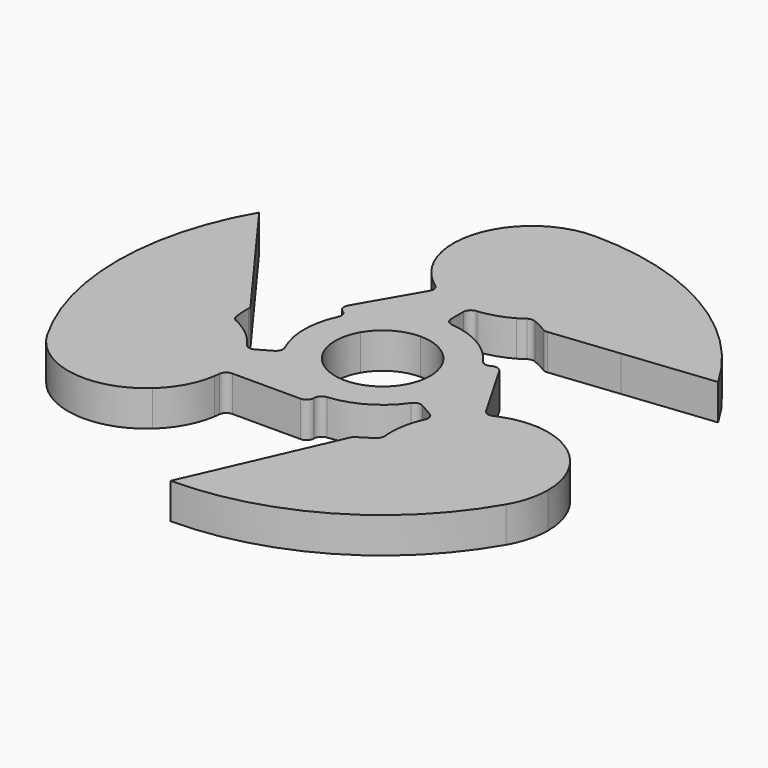
from build123d import *

# Parameters (mm, degrees)
F1_DEPTH = 4.7625
F2_R     = 1


with BuildPart() as f1:
    # F0 (on Top) → F1 (new body)
    with BuildSketch(Plane.XY):
        with BuildLine():
            ThreePointArc((-5.499261314, -3.175), (-6.35, 0), (-5.499261314, 3.175))
            Line((-5.499261314, 3.175), (-9.0932667397, 5.25))
            ThreePointArc((-9.0932667397, 5.25), (-10.5, 0), (-9.0932667397, -5.25))
            Line((-9.0932667397, -5.25), (-5.499261314, -3.175))
        make_face()
        with BuildLine():
            Line((0, -10.5), (0, -6.35))
            ThreePointArc((0, -6.35), (-3.175, -5.499261314), (-5.499261314, -3.175))
            Line((-5.499261314, -3.175), (-9.0932667397, -5.25))
            ThreePointArc((-9.0932667397, -5.25), (-5.25, -9.0932667397), (0, -10.5))
        make_face()
        with BuildLine():
            Line((9.0932667397, -5.25), (5.499261314, -3.175))
            ThreePointArc((5.499261314, -3.175), (3.175, -5.499261314), (0, -6.35))
            Line((0, -6.35), (0, -10.5))
            ThreePointArc((0, -10.5), (5.25, -9.0932667397), (9.0932667397, -5.25))
        make_face()
        with BuildLine():
            ThreePointArc((5.499261314, 3.175), (6.1336289969, 1.6435009364), (6.35, 0))
            ThreePointArc((6.35, 0), (6.1336289969, -1.6435009364), (5.499261314, -3.175))
            Line((5.499261314, -3.175), (9.0932667397, -5.25))
            ThreePointArc((9.0932667397, -5.25), (10.142221176, -2.7175999736), (10.5, 0))
            ThreePointArc((10.5, 0), (10.142221176, 2.7175999736), (9.0932667397, 5.25))
            Line((9.0932667397, 5.25), (5.499261314, 3.175))
        make_face()
        with BuildLine():
            ThreePointArc((0, 6.35), (3.175, 5.499261314), (5.499261314, 3.175))
            Line((5.499261314, 3.175), (9.0932667397, 5.25))
            ThreePointArc((9.0932667397, 5.25), (5.25, 9.0932667397), (0, 10.5))
            Line((0, 10.5), (0, 6.35))
        make_face()
        with BuildLine():
            ThreePointArc((-5.499261314, 3.175), (-3.175, 5.499261314), (0, 6.35))
            Line((0, 6.35), (0, 10.5))
            ThreePointArc((0, 10.5), (-5.25, 9.0932667397), (-9.0932667397, 5.25))
            Line((-9.0932667397, 5.25), (-5.499261314, 3.175))
        make_face()
        with BuildLine():
            Line((-30.6832667397, -17.7149923118), (-21.59, -12.4649923118))
            ThreePointArc((-21.59, -12.4649923118), (-23.7308339091, -7.638825519), (-24.8073171849, -2.4700500843))
            ThreePointArc((-24.8073171849, -2.4700500843), (-31.387432573, -8.6887090891), (-30.6832667397, -17.7149923118))
        make_face()
        with BuildLine():
            ThreePointArc((-14.5427847141, -20.2487418398), (-18.4808339091, -16.7320922588), (-21.59, -12.4649923118))
            Line((-21.59, -12.4649923118), (-30.6832667397, -17.7149923118))
            ThreePointArc((-30.6832667397, -17.7149923118), (-23.2183590837, -22.8379594232), (-14.5427847141, -20.2487418398))
        make_face()
        with BuildLine():
            ThreePointArc((-24.8073171849, -2.4700500843), (-24.7664239313, 2.8510312146), (-23.5971783755, 8.0422202188))
            Line((-23.5971783755, 8.0422202188), (-30.6832667397, 17.7149923118))
            ThreePointArc((-30.6832667397, 17.7149923118), (-35.4299846236, 0), (-30.6832667397, -17.7149923118))
            ThreePointArc((-30.6832667397, -17.7149923118), (-31.387432573, -8.6887090891), (-24.8073171849, -2.4700500843))
        make_face()
        with BuildLine():
            ThreePointArc((-17.8004721403, -2.6726749865), (-17.9637015789, -1.1425522236), (-17.9956452163, 0.3959207605))
            Line((-17.9956452163, 0.3959207605), (-23.5971783755, 8.0422202188))
            ThreePointArc((-23.5971783755, 8.0422202188), (-24.7664239313, 2.8510312146), (-24.8073171849, -2.4700500843))
            ThreePointArc((-24.8073171849, -2.4700500843), (-21.286486447, -1.9693799179), (-17.8004721403, -2.6726749865))
        make_face()
        with BuildLine():
            Line((-21.59, -12.4649923118), (-17.2877645627, -5.0133019483))
            ThreePointArc((-17.2877645627, -5.0133019483), (-17.5831090076, -3.851529258), (-17.8004721403, -2.6726749865))
            ThreePointArc((-17.8004721403, -2.6726749865), (-21.286486447, -1.9693799179), (-24.8073171849, -2.4700500843))
            ThreePointArc((-24.8073171849, -2.4700500843), (-23.7308339091, -7.638825519), (-21.59, -12.4649923118))
        make_face()
        with BuildLine():
            ThreePointArc((-11.2148405045, -14.0793235796), (-12.1270766847, -13.3016544491), (-12.9855291254, -12.4649923118))
            Line((-12.9855291254, -12.4649923118), (-21.59, -12.4649923118))
            ThreePointArc((-21.59, -12.4649923118), (-18.4808339091, -16.7320922588), (-14.5427847141, -20.2487418398))
            ThreePointArc((-14.5427847141, -20.2487418398), (-12.3487762621, -17.4499480615), (-11.2148405045, -14.0793235796))
        make_face()
        with BuildLine():
            ThreePointArc((-12.9855291254, -12.4649923118), (-14.3916544405, -10.8111184651), (-15.5884572681, -9))
            Line((-15.5884572681, -9), (-21.59, -12.4649923118))
            Line((-21.59, -12.4649923118), (-12.9855291254, -12.4649923118))
        make_face()
        with BuildLine():
            Line((-21.59, -12.4649923118), (-15.5884572681, -9))
            ThreePointArc((-15.5884572681, -9), (-16.5585304543, -7.0579791154), (-17.2877645627, -5.0133019483))
            Line((-17.2877645627, -5.0133019483), (-21.59, -12.4649923118))
        make_face()
        with BuildLine():
            Line((-15.5884572681, -9), (-12.4967332603, -7.2149923118))
            ThreePointArc((-12.4967332603, -7.2149923118), (-12.8045182874, -6.7147478755), (-13.139793395, -6.2324961559))
            ThreePointArc((-13.139793395, -6.2324961559), (-14.5921490915, -4.6368327157), (-16.34, -3.3717255721))
            Line((-16.34, -3.3717255721), (-17.2877645627, -5.0133019483))
            ThreePointArc((-17.2877645627, -5.0133019483), (-16.5585304543, -7.0579791154), (-15.5884572681, -9))
        make_face()
        with BuildLine():
            ThreePointArc((-11.09, -12.4649923118), (-11.447778824, -9.7473923382), (-12.4967332603, -7.2149923118))
            Line((-12.4967332603, -7.2149923118), (-15.5884572681, -9))
            ThreePointArc((-15.5884572681, -9), (-14.3916544405, -10.8111184651), (-12.9855291254, -12.4649923118))
            Line((-12.9855291254, -12.4649923118), (-11.09, -12.4649923118))
        make_face()
        with BuildLine():
            Line((-17.2877645627, -5.0133019483), (-16.34, -3.3717255721))
            ThreePointArc((-16.34, -3.3717255721), (-17.0567413584, -2.9940068252), (-17.8004721403, -2.6726749865))
            ThreePointArc((-17.8004721403, -2.6726749865), (-17.5831090076, -3.851529258), (-17.2877645627, -5.0133019483))
        make_face()
        with BuildLine():
            ThreePointArc((-11.2148405045, -14.0793235796), (-11.1212566489, -13.2745679095), (-11.09, -12.4649923118))
            Line((-11.09, -12.4649923118), (-12.9855291254, -12.4649923118))
            ThreePointArc((-12.9855291254, -12.4649923118), (-12.1270766847, -13.3016544491), (-11.2148405045, -14.0793235796))
        make_face()
        with BuildLine():
            Line((21.59, -12.4649923118), (17.2877645627, -5.0133019483))
            ThreePointArc((17.2877645627, -5.0133019483), (16.5585304543, -7.0579791154), (15.5884572681, -9))
            Line((15.5884572681, -9), (21.59, -12.4649923118))
        make_face()
        with BuildLine():
            Line((17.2877645627, -5.0133019483), (16.34, -3.3717255721))
            ThreePointArc((16.34, -3.3717255721), (14.1653787975, -5.0403711093), (12.4967332603, -7.2149923118))
            Line((12.4967332603, -7.2149923118), (15.5884572681, -9))
            ThreePointArc((15.5884572681, -9), (16.5585304543, -7.0579791154), (17.2877645627, -5.0133019483))
        make_face()
        with BuildLine():
            Line((15.5884572681, -9), (12.4967332603, -7.2149923118))
            ThreePointArc((12.4967332603, -7.2149923118), (12.2250524559, -7.7165444079), (11.9810090739, -8.2321099153))
            ThreePointArc((11.9810090739, -8.2321099153), (11.3151665531, -10.3021706275), (11.09, -12.4649923118))
            Line((11.09, -12.4649923118), (12.9855291254, -12.4649923118))
            ThreePointArc((12.9855291254, -12.4649923118), (14.3916544405, -10.8111184651), (15.5884572681, -9))
        make_face()
        with BuildLine():
            Line((21.59, -12.4649923118), (15.5884572681, -9))
            ThreePointArc((15.5884572681, -9), (14.3916544405, -10.8111184651), (12.9855291254, -12.4649923118))
            Line((12.9855291254, -12.4649923118), (21.59, -12.4649923118))
        make_face()
        with BuildLine():
            ThreePointArc((14.5427847141, -20.2487418398), (18.4808339091, -16.7320922588), (21.59, -12.4649923118))
            Line((21.59, -12.4649923118), (12.9855291254, -12.4649923118))
            ThreePointArc((12.9855291254, -12.4649923118), (12.1270766847, -13.3016544491), (11.2148405045, -14.0793235796))
            ThreePointArc((11.2148405045, -14.0793235796), (12.3487762621, -17.4499480615), (14.5427847141, -20.2487418398))
        make_face()
        with BuildLine():
            ThreePointArc((24.8073171849, -2.4700500843), (23.7308339091, -7.638825519), (21.59, -12.4649923118))
            Line((21.59, -12.4649923118), (30.6832667397, -17.7149923118))
            ThreePointArc((30.6832667397, -17.7149923118), (31.732221176, -15.1825922854), (32.09, -12.4649923118))
            ThreePointArc((32.09, -12.4649923118), (30.0762191358, -6.2816206766), (24.8073171849, -2.4700500843))
        make_face()
        with BuildLine():
            ThreePointArc((17.8004721403, -2.6726749865), (17.5831090076, -3.851529258), (17.2877645627, -5.0133019483))
            Line((17.2877645627, -5.0133019483), (21.59, -12.4649923118))
            ThreePointArc((21.59, -12.4649923118), (23.7308339091, -7.638825519), (24.8073171849, -2.4700500843))
            ThreePointArc((24.8073171849, -2.4700500843), (21.286486447, -1.9693799179), (17.8004721403, -2.6726749865))
        make_face()
        with BuildLine():
            ThreePointArc((17.8004721403, -2.6726749865), (17.0567413584, -2.9940068252), (16.34, -3.3717255721))
            Line((16.34, -3.3717255721), (17.2877645627, -5.0133019483))
            ThreePointArc((17.2877645627, -5.0133019483), (17.5831090076, -3.851529258), (17.8004721403, -2.6726749865))
        make_face()
        with BuildLine():
            ThreePointArc((30.6832667397, -17.7149923118), (23.2183590837, -22.8379594232), (14.5427847141, -20.2487418398))
            ThreePointArc((14.5427847141, -20.2487418398), (9.9141341412, -22.8738732523), (4.8337957326, -24.4568712666))
            Line((4.8337957326, -24.4568712666), (0, -35.4299846236))
            ThreePointArc((0, -35.4299846236), (17.7149923118, -30.6832667397), (30.6832667397, -17.7149923118))
        make_face()
        with BuildLine():
            ThreePointArc((11.2148405045, -14.0793235796), (9.9713029836, -14.9857638047), (8.6548881807, -15.7826775479))
            Line((8.6548881807, -15.7826775479), (4.8337957326, -24.4568712666))
            ThreePointArc((4.8337957326, -24.4568712666), (9.9141341412, -22.8738732523), (14.5427847141, -20.2487418398))
            ThreePointArc((14.5427847141, -20.2487418398), (12.3487762621, -17.4499480615), (11.2148405045, -14.0793235796))
        make_face()
        with BuildLine():
            Line((12.9855291254, -12.4649923118), (11.09, -12.4649923118))
            ThreePointArc((11.09, -12.4649923118), (11.1212566489, -13.2745679095), (11.2148405045, -14.0793235796))
            ThreePointArc((11.2148405045, -14.0793235796), (12.1270766847, -13.3016544491), (12.9855291254, -12.4649923118))
        make_face()
        with BuildLine():
            Line((30.6832667397, -17.7149923118), (21.59, -12.4649923118))
            ThreePointArc((21.59, -12.4649923118), (18.4808339091, -16.7320922588), (14.5427847141, -20.2487418398))
            ThreePointArc((14.5427847141, -20.2487418398), (23.2183590837, -22.8379594232), (30.6832667397, -17.7149923118))
        make_face()
        with BuildLine():
            Line((0, 18), (0, 14.4299846236))
            ThreePointArc((0, 14.4299846236), (0.5701972901, 14.4454781951), (1.1387118387, 14.4919131854))
            ThreePointArc((1.1387118387, 14.4919131854), (3.2643582308, 14.9503070065), (5.25, 15.8367178839))
            Line((5.25, 15.8367178839), (4.3022354373, 17.4782942601))
            ThreePointArc((4.3022354373, 17.4782942601), (2.1668760138, 17.8690975805), (0, 18))
        make_face()
        with BuildLine():
            ThreePointArc((-4.3022354373, 17.4782942601), (-2.1668760138, 17.8690975805), (0, 18))
            Line((0, 18), (0, 24.9299846236))
            Line((0, 24.9299846236), (-4.3022354373, 17.4782942601))
        make_face()
        with BuildLine():
            Line((0, 24.9299846236), (0, 18))
            ThreePointArc((0, 18), (2.1668760138, 17.8690975805), (4.3022354373, 17.4782942601))
            Line((4.3022354373, 17.4782942601), (0, 24.9299846236))
        make_face()
        with BuildLine():
            ThreePointArc((-6.5856316358, 16.7519985661), (-5.9354847095, 16.2685747347), (-5.25, 15.8367178839))
            Line((-5.25, 15.8367178839), (-4.3022354373, 17.4782942601))
            ThreePointArc((-4.3022354373, 17.4782942601), (-5.456032323, 17.1531837071), (-6.5856316358, 16.7519985661))
        make_face()
        with BuildLine():
            Line((0, 24.9299846236), (4.3022354373, 17.4782942601))
            ThreePointArc((4.3022354373, 17.4782942601), (5.456032323, 17.1531837071), (6.5856316358, 16.7519985661))
            ThreePointArc((6.5856316358, 16.7519985661), (8.9377101849, 19.4193279794), (10.2645324709, 22.718791924))
            ThreePointArc((10.2645324709, 22.718791924), (5.25, 24.3709177778), (0, 24.9299846236))
        make_face()
        with BuildLine():
            Line((4.3022354373, 17.4782942601), (5.25, 15.8367178839))
            ThreePointArc((5.25, 15.8367178839), (5.9354847095, 16.2685747347), (6.5856316358, 16.7519985661))
            ThreePointArc((6.5856316358, 16.7519985661), (5.456032323, 17.1531837071), (4.3022354373, 17.4782942601))
        make_face()
        with BuildLine():
            ThreePointArc((-5.25, 15.8367178839), (-2.7175999736, 14.7877634476), (0, 14.4299846236))
            Line((0, 14.4299846236), (0, 18))
            ThreePointArc((0, 18), (-2.1668760138, 17.8690975805), (-4.3022354373, 17.4782942601))
            Line((-4.3022354373, 17.4782942601), (-5.25, 15.8367178839))
        make_face()
        with BuildLine():
            ThreePointArc((-6.5856316358, 16.7519985661), (-5.456032323, 17.1531837071), (-4.3022354373, 17.4782942601))
            Line((-4.3022354373, 17.4782942601), (0, 24.9299846236))
            ThreePointArc((0, 24.9299846236), (-5.25, 24.3709177778), (-10.2645324709, 22.718791924))
            ThreePointArc((-10.2645324709, 22.718791924), (-8.9377101849, 19.4193279794), (-6.5856316358, 16.7519985661))
        make_face()
        with BuildLine():
            ThreePointArc((-10.2645324709, 22.718791924), (-5.25, 24.3709177778), (0, 24.9299846236))
            Line((0, 24.9299846236), (0, 35.4299846236))
            ThreePointArc((0, 35.4299846236), (-8.1690734892, 31.5266685123), (-10.2645324709, 22.718791924))
        make_face()
        with BuildLine():
            Line((0, 35.4299846236), (0, 24.9299846236))
            ThreePointArc((0, 24.9299846236), (5.25, 24.3709177778), (10.2645324709, 22.718791924))
            ThreePointArc((10.2645324709, 22.718791924), (10.4409671713, 23.8181372744), (10.5, 24.9299846236))
            ThreePointArc((10.5, 24.9299846236), (7.4246212025, 32.3546058261), (0, 35.4299846236))
        make_face()
        with BuildLine():
            ThreePointArc((10.2645324709, 22.718791924), (14.8522882489, 20.022828649), (18.7633739476, 16.4146255344))
            Line((18.7633739476, 16.4146255344), (30.6832667397, 17.7149923118))
            ThreePointArc((30.6832667397, 17.7149923118), (17.7149923118, 30.6832667397), (0, 35.4299846236))
            ThreePointArc((0, 35.4299846236), (7.4246212025, 32.3546058261), (10.5, 24.9299846236))
            ThreePointArc((10.5, 24.9299846236), (10.4409671713, 23.8181372744), (10.2645324709, 22.718791924))
        make_face()
        with BuildLine():
            ThreePointArc((6.5856316358, 16.7519985661), (7.9924006582, 16.128283595), (9.3407556058, 15.3866918053))
            Line((9.3407556058, 15.3866918053), (18.7633739476, 16.4146255344))
            ThreePointArc((18.7633739476, 16.4146255344), (14.8522882489, 20.022828649), (10.2645324709, 22.718791924))
            ThreePointArc((10.2645324709, 22.718791924), (8.9377101849, 19.4193279794), (6.5856316358, 16.7519985661))
        make_face()
        with BuildLine():
            ThreePointArc((-9.0932667397, 5.25), (-5.25, 9.0932667397), (0, 10.5))
            Line((0, 10.5), (0, 14.3676886584))
            Line((0, 14.3676886584), (0, 14.4299846236))
            ThreePointArc((0, 14.4299846236), (-2.7175999736, 14.7877634476), (-5.25, 15.8367178839))
            Line((-5.25, 15.8367178839), (-10.795, 6.2324961559))
            Line((-10.795, 6.2324961559), (-9.0932667397, 5.25))
        make_face()
        with BuildLine():
            Line((10.795, 6.2324961559), (9.0932667397, 5.25))
            ThreePointArc((9.0932667397, 5.25), (10.142221176, 2.7175999736), (10.5, 0))
            ThreePointArc((10.5, 0), (10.142221176, -2.7175999736), (9.0932667397, -5.25))
            Line((9.0932667397, -5.25), (12.4427833719, -7.1838443292))
            Line((12.4427833719, -7.1838443292), (12.4967332603, -7.2149923118))
            ThreePointArc((12.4967332603, -7.2149923118), (14.1653787975, -5.0403711093), (16.34, -3.3717255721))
            Line((16.34, -3.3717255721), (10.795, 6.2324961559))
        make_face()
        with BuildLine():
            Line((0, -12.4649923118), (0, -10.5))
            ThreePointArc((0, -10.5), (-5.25, -9.0932667397), (-9.0932667397, -5.25))
            Line((-9.0932667397, -5.25), (-12.4967332603, -7.2149923118))
            ThreePointArc((-12.4967332603, -7.2149923118), (-11.447778824, -9.7473923382), (-11.09, -12.4649923118))
            Line((-11.09, -12.4649923118), (0, -12.4649923118))
        make_face()
    extrude(amount=F1_DEPTH)

    # F2
    f2_edges = [f1.edges().sort_by_distance(p)[0] for p in [
        (0, -12.464992, 2.38125),
        (10.795, 6.232496, 2.38125),
        (-10.795, 6.232496, 2.38125),
        (8.654888, -15.782678, 2.38125),
        (11.214841, -14.079324, 2.38125),
        (-17.995645, 0.395921, 2.38125),
        (-17.800472, -2.672675, 2.38125),
        (9.340756, 15.386692, 2.38125),
        (6.585632, 16.751999, 2.38125),
        (0, 35.429985, 2.38125),
        (9.093267, -5.25, 2.38125),
        (0, -10.5, 2.38125),
        (0, 10.5, 2.38125),
        (-9.093267, -5.25, 2.38125),
        (30.683267, -17.714992, 2.38125),
        (-9.093267, 5.25, 2.38125),
        (-5.25, 15.836718, 2.38125),
        (-11.09, -12.464992, 2.38125),
        (9.093267, 5.25, 2.38125),
        (-30.683267, -17.714992, 2.38125),
        (16.34, -3.371726, 2.38125),
        (-12.496733, -7.214992, 2.38125),
        (12.496733, -7.214992, 2.38125),
        (0, 14.429985, 2.38125),
    ]]
    fillet(f2_edges, radius=F2_R)


solid = f1.part
